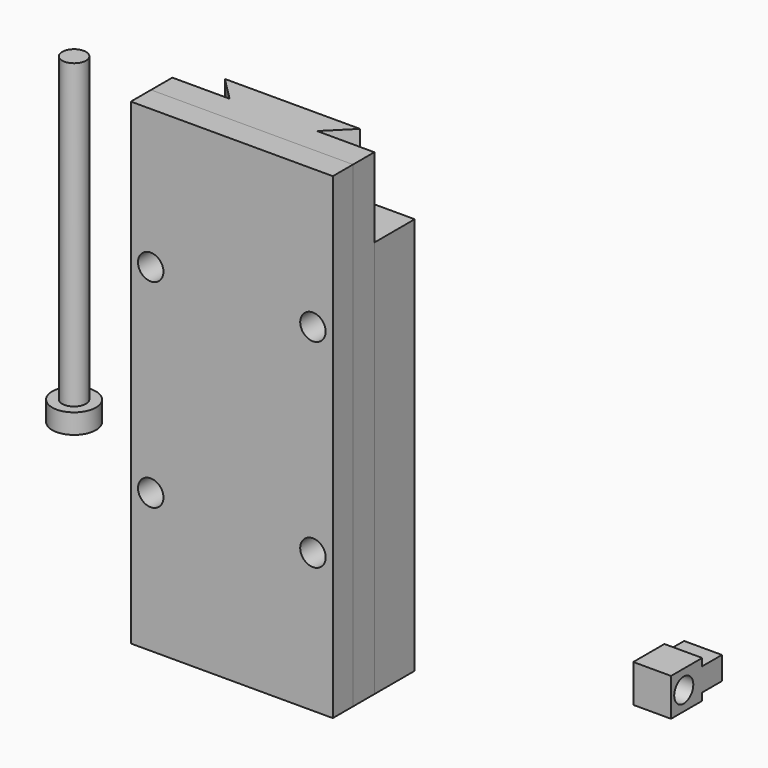
from build123d import *

# Parameters (mm, degrees)
F1_DEPTH  = 60
F2_W      = 3.2
F2_H      = 42
F3_DEPTH  = 3.5
F4_W      = 8
F4_H      = 7.5
F5_DEPTH  = 6.351
F6_W      = 5
F6_H      = 21
F7_DEPTH  = 5
F8_R      = 2.75
F9_DEPTH  = 2.5
F10_R     = 1.5
F11_DEPTH = 38
F13_R     = 4
F13_R_2   = 1.5
F14_DEPTH = 4
F15_DEPTH = 2
F16_W     = 3
F16_H     = 17
F17_DEPTH = 28.3600109795
F18_R     = 1.25
F19_DEPTH = 3.35
F20_W     = 25.4
F20_H     = 60
F20_R     = 1.6
F21_DEPTH = 3.175
F23_DEPTH = 50
F24_W     = 4.75
F24_H     = 8
F25_DEPTH = 4.75
F26_R     = 1.5
F27_DEPTH = 87.9577198902
F28_W     = 3.1
F28_H     = 0.925
F29_DEPTH = 87.9577198902


# Not quite as in the source:
# - a length typed as a fraction of an inch, garbled in the dataset ("3 / 203.2 mm" for 3/8 in), is restored


with BuildPart() as f1:
    # F0 (on Top) → F1 (new body)
    with BuildSketch(Plane.XY):
        Polygon((-12.7, 3.35), (-12.7, 0), (12.7, 0), (12.7, 3.35), (5.5, 3.35), (8.5, 6.35), (-8.5, 6.35), (-5.5, 3.35), align=None)
    extrude(amount=F1_DEPTH)

    # F2 (on face) → F3 (cut)
    with BuildSketch(Plane.XZ):
        with Locations((0, 21)):
            Rectangle(F2_W, F2_H)
    extrude(amount=-F3_DEPTH, mode=Mode.SUBTRACT)

    # F4 (on face) → F5 (cut, through all)
    with BuildSketch(Plane.XZ):
        with Locations((0, 38.25)):
            Rectangle(F4_W, F4_H)
        with Locations((0, 3.75)):
            Rectangle(F4_W, F4_H)
    extrude(amount=-F5_DEPTH, mode=Mode.SUBTRACT)

    # F6 (on face) → F7 (cut)
    with BuildSketch(Plane.XZ):
        with Locations((0, 21)):
            Rectangle(F6_W, F6_H)
    extrude(amount=-F7_DEPTH, mode=Mode.SUBTRACT)

    # F16 (on face) → F17 (cut, through all)
    with BuildSketch(Plane.XZ.offset(-5)):
        with Locations((0, 21)):
            Rectangle(F16_W, F16_H)
    extrude(amount=-F17_DEPTH, mode=Mode.SUBTRACT)

    # F18 (on face) → F19 (cut, through all)
    with BuildSketch(Plane.XZ):
        with Locations((10.2, 17.5)):
            Circle(F18_R)
        with Locations((-10.2, 17.5)):
            Circle(F18_R)
        with Locations((10.2, 42.5)):
            Circle(F18_R)
        with Locations((-10.2, 42.5)):
            Circle(F18_R)
    extrude(amount=-F19_DEPTH, mode=Mode.SUBTRACT)


with BuildPart() as f9:
    # F8 (on Top) → F9 (new body)
    with BuildSketch(Plane.XY):
        with Locations((-46.4769527316, 30.1239509135)):
            Circle(F8_R)
    extrude(amount=F9_DEPTH)

    # F10 (on face) → F11 (join)
    with BuildSketch(Plane.XY.offset(2.5)):
        with Locations((-46.4769527316, 30.1239509135)):
            Circle(F10_R)
    extrude(amount=F11_DEPTH)

    # F12 (on face) → F15 (cut)
    with BuildSketch(Plane(origin=(0, 0, 0), x_dir=(1, 0, 0), z_dir=(0, 0, -1))):
        Polygon((-46.7203685833, -28.7012485355), (-47.8307570588, -29.6234040357), (-47.5873412072, -31.0461064138), (-46.23353688, -31.5466532916), (-45.1231484044, -30.6244977914), (-45.366564256, -29.2017954133), align=None)
    extrude(amount=-F15_DEPTH, mode=Mode.SUBTRACT)


with BuildPart() as f14:
    # F13 (on Top) → F14 (new body)
    with BuildSketch(Plane.XY):
        with Locations((-21.5977616608, 29.3590109795)):
            Circle(F13_R)
        with Locations((-21.5977616608, 29.3590109795)):
            Circle(F13_R_2, mode=Mode.SUBTRACT)
    extrude(amount=F14_DEPTH)


with BuildPart() as f21:
    # F20 (on face) → F21 (new body)
    with BuildSketch(Plane.XZ):
        with Locations((0, 30)):
            Rectangle(F20_W, F20_H)
        with Locations((-10.2, 17.5)):
            Circle(F20_R, mode=Mode.SUBTRACT)
        with Locations((10.2, 17.5)):
            Circle(F20_R, mode=Mode.SUBTRACT)
        with Locations((-10.2, 42.5)):
            Circle(F20_R, mode=Mode.SUBTRACT)
        with Locations((10.2, 42.5)):
            Circle(F20_R, mode=Mode.SUBTRACT)
    extrude(amount=F21_DEPTH)


with BuildPart() as f23:
    # F22 (on Top) → F23 (new body)
    with BuildSketch(Plane.XY):
        Polygon((12.7, 9.7), (-12.7, 9.7), (-12.7, 3.35), (-5.5, 3.35), (-8.5, 6.35), (8.5, 6.35), (5.5, 3.35), (12.7, 3.35), align=None)
    extrude(amount=F23_DEPTH)


with BuildPart() as f25:
    # F24 (on Top) → F25 (new body)
    with BuildSketch(Plane.XY):
        with Locations((36.3547671586, 21.4546729288)):
            Rectangle(F24_W, F24_H)
    extrude(amount=F25_DEPTH)

    # F26 (on face) → F27 (cut, through all)
    with BuildSketch(Plane.YZ.offset(38.7297671586)):
        with Locations((19.4546729288, 2.375)):
            Circle(F26_R)
    extrude(amount=-F27_DEPTH, mode=Mode.SUBTRACT)

    # F28 (on face) → F29 (cut, through all)
    with BuildSketch(Plane.YZ.offset(38.7297671586)):
        with Locations((23.9046729288, 4.2875)):
            Rectangle(F28_W, F28_H)
        with Locations((23.9046729288, 0.4625)):
            Rectangle(F28_W, F28_H)
    extrude(amount=-F29_DEPTH, mode=Mode.SUBTRACT)


solid = Compound([f1.part, f9.part, f14.part, f21.part, f23.part, f25.part])
